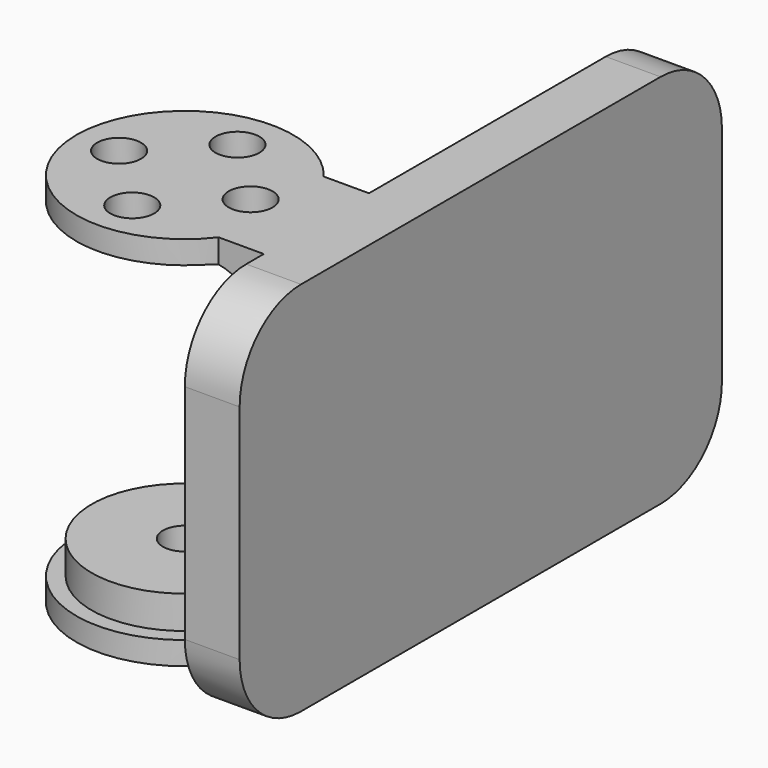
from build123d import *

# Parameters (mm, degrees)
F1_DEPTH      = 17.15
F3_DEPTH      = 40.001
F3_DEPTH_BACK = 15.001
F5_R          = 8.5
F6_DEPTH      = 3
F7_R          = 2
F8_DEPTH      = 5.1010001
F9_R          = 2
F10_DEPTH     = 17.15
F11_R         = 7


with BuildPart() as f1:
    # F0 (on Top) → F1 (new body)
    with BuildSketch(Plane.XY):
        with BuildLine():
            Line((12, 6), (7.874642849, 6))
            ThreePointArc((7.874642849, 6), (-9.9, 0), (7.874642849, -6))
            Line((7.874642849, -6), (12, -6))
            Line((12, -6), (12, -15))
            Line((12, -15), (17, -15))
            Line((17, -15), (17, 40))
            Line((17, 40), (12, 40))
            Line((12, 40), (12, 6))
        make_face()
    extrude(amount=F1_DEPTH)

    # F2 (on Front) → F3 (cut, two sides)
    with BuildSketch(Plane.XZ) as f3_sk:
        with BuildLine():
            Line((7, 15.05), (-20, 15.05))
            Line((-20, 15.05), (-20, 0))
            Line((-20, 0), (12, 0))
            Line((12, 0), (12, 10.05))
            ThreePointArc((12, 10.05), (10.5355339059, 13.5855339059), (7, 15.05))
        make_face()
    extrude(amount=-F3_DEPTH, mode=Mode.SUBTRACT)
    extrude(f3_sk.sketch, amount=F3_DEPTH_BACK, mode=Mode.SUBTRACT)

    # F4: F1 across plane


with BuildPart() as f1_1:
    add(f1.part)
    add(f1.part.mirror(Plane.XY))

    # F5 (on face) → F6 (join)
    with BuildSketch(Plane.XY.offset(-15.05)):
        Circle(F5_R)
    extrude(amount=F6_DEPTH)

    # F7 (on face) → F8 (cut, through all)
    with BuildSketch(Plane.XY.offset(-12.05)):
        Circle(F7_R)
    extrude(amount=-F8_DEPTH, mode=Mode.SUBTRACT)

    # F9 (on face) → F10 (cut, through all)
    with BuildSketch(Plane.XY.offset(17.15)):
        with Locations((6, 0)):
            Circle(F9_R)
        with Locations((0, -6)):
            Circle(F9_R)
        with Locations((-6, 0)):
            Circle(F9_R)
        with Locations((0, 6)):
            Circle(F9_R)
    extrude(amount=-F10_DEPTH, mode=Mode.SUBTRACT)

    # F11
    f11_edges = [f1_1.edges().sort_by_distance(p)[0] for p in [
        (14.5, 40, 17.15),
        (14.5, 40, -17.15),
        (14.5, -15, -17.15),
        (14.5, -15, 17.15),
    ]]
    fillet(f11_edges, radius=F11_R)


solid = f1_1.part
